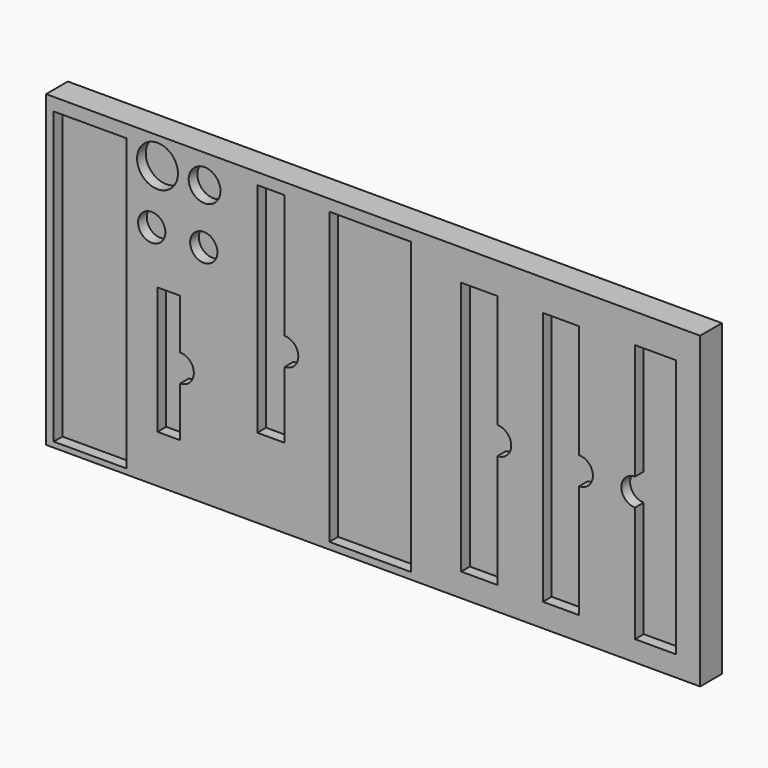
from build123d import *

# Parameters (mm, degrees)
F0_W     = 457.2
F0_H     = 215.9
F1_DEPTH = 19.05
F2_W     = 50.8
F2_H     = 203.2
F2_W_2   = 15.875
F2_H_2   = 88.9
F2_W_3   = 19.05
F2_H_3   = 152.4
F2_W_4   = 57.15
F2_W_5   = 25.4
F2_H_4   = 177.8
F2_W_6   = 28.575
F2_H_5   = 180.975
F2_R     = 14.2875
F2_R_2   = 11.1125
F2_R_3   = 9.525
F3_DEPTH = 7.62
F5_DEPTH = 7.62


# Not quite as in the source:
# - a length typed as a fraction of an inch, garbled in the dataset ("3 / 203.2 mm" for 3/8 in), is restored


with BuildPart() as f1:
    # F0 (on Front) → F1 (new body)
    with BuildSketch(Plane.XZ):
        with Locations((34.5792232292, 7.7549852431)):
            Rectangle(F0_W, F0_H)
    extrude(amount=F1_DEPTH)

    # F2 (on face) → F3 (cut)
    with BuildSketch(Plane.XZ.offset(19.05)):
        with Locations((-163.2603832245, 5.173290801)):
            Rectangle(F2_W, F2_H)
        with Locations((-108.1939504743, -22.3739650816)):
            Rectangle(F2_W_2, F2_H_2)
        with Locations((-36.7521092981, 31.5419817448)):
            Rectangle(F2_W_3, F2_H_3)
        with Locations((32.6018253148, 6.1419817448)):
            Rectangle(F2_W_4, F2_H)
        with Locations((108.8770244598, 5.1134674311)):
            Rectangle(F2_W_5, F2_H_4)
        with Locations((165.9826848984, 5.1134674311)):
            Rectangle(F2_W_5, F2_H_4)
        with Locations((231.9335953236, 4.6242426157)):
            Rectangle(F2_W_6, F2_H_5)
        with Locations((-116.1314504743, 96.762670864)):
            Circle(F2_R)
        with Locations((-83.2345709205, 95.660790801)):
            Circle(F2_R_2)
        with Locations((-83.7836638093, 57.2242997587)):
            Circle(F2_R_3)
        with Locations((-120.1787297428, 57.6790883665)):
            Circle(F2_R_3)
    extrude(amount=-F3_DEPTH, mode=Mode.SUBTRACT)

    # F4 (on face) → F5 (cut)
    with BuildSketch(Plane.XZ.offset(19.05)):
        with BuildLine():
            ThreePointArc((-100.2564504743, -31.8989650816), (-93.5212583835, -29.1091571724), (-90.7314504743, -22.3739650816))
            ThreePointArc((-90.7314504743, -22.3739650816), (-93.5212583835, -15.6387729908), (-100.2564504743, -12.8489650816))
            Line((-100.2564504743, -12.8489650816), (-100.2564504743, -31.8989650816))
        make_face()
        with BuildLine():
            ThreePointArc((-27.2271092981, 2.0650514647), (-20.4919172073, 4.8548593739), (-17.7021092981, 11.5900514647))
            ThreePointArc((-17.7021092981, 11.5900514647), (-20.4919172073, 18.3252435555), (-27.2271092981, 21.1150514647))
            Line((-27.2271092981, 21.1150514647), (-27.2271092981, 2.0650514647))
        make_face()
        with BuildLine():
            ThreePointArc((121.5770244598, -4.4115325689), (128.3122165506, -1.6217246597), (131.1020244598, 5.1134674311))
            ThreePointArc((131.1020244598, 5.1134674311), (128.3122165506, 11.8486595219), (121.5770244598, 14.6384674311))
            Line((121.5770244598, 14.6384674311), (121.5770244598, -4.4115325689))
        make_face()
        with BuildLine():
            ThreePointArc((178.6826848984, -4.4115325689), (185.4178769892, -1.6217246597), (188.2076848984, 5.1134674311))
            ThreePointArc((188.2076848984, 5.1134674311), (185.4178769892, 11.8486595219), (178.6826848984, 14.6384674311))
            Line((178.6826848984, 14.6384674311), (178.6826848984, -4.4115325689))
        make_face()
        with BuildLine():
            ThreePointArc((217.6460953236, -4.9007573843), (224.3812874144, -2.1109494751), (227.1710953236, 4.6242426157))
            ThreePointArc((227.1710953236, 4.6242426157), (224.3812874144, 11.3594347065), (217.6460953236, 14.1492426157))
            Line((217.6460953236, 14.1492426157), (217.6460953236, -4.9007573843))
        make_face()
        with BuildLine():
            Line((217.6460953236, -4.9007573843), (217.6460953236, 14.1492426157))
            ThreePointArc((217.6460953236, 14.1492426157), (208.1210953236, 4.6242426157), (217.6460953236, -4.9007573843))
        make_face()
    extrude(amount=-F5_DEPTH, mode=Mode.SUBTRACT)


solid = f1.part
